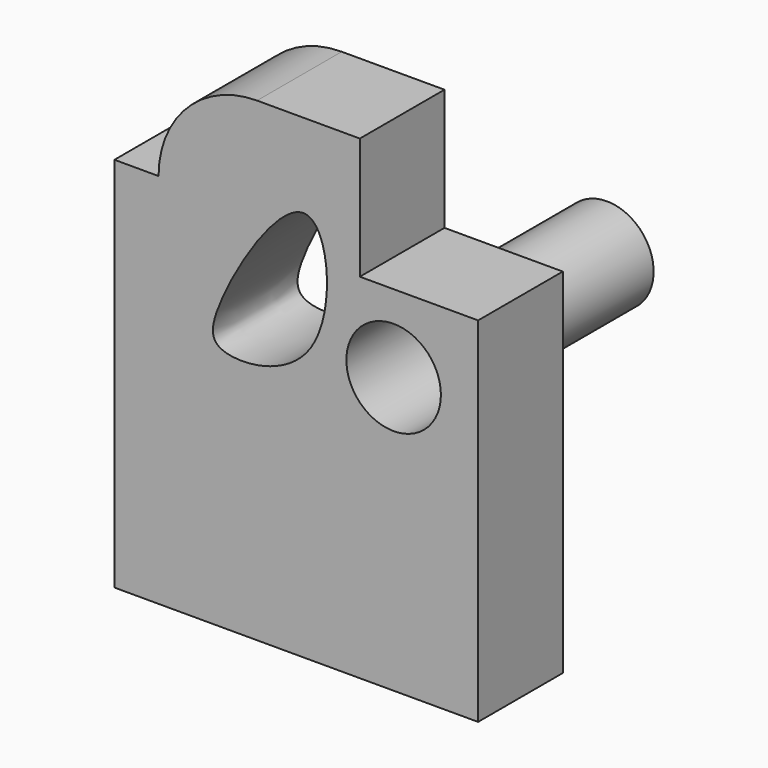
from build123d import *

# Parameters (mm, degrees)
F0_R      = 27.2043930804
F1_DEPTH  = 60.893477872
F2_R      = 56.6833195886
F3_R      = 26.9202980766
F4_DEPTH  = 188.1199926138
F5_DEPTH  = 143.7802445143
F8_DEPTH  = 25.4
F9_DEPTH  = 88.3794147521
F10_DEPTH = 95.6057533622


# Not quite as in the source:
# - a feature of the source that left no trace in its solid (it failed there, or was rolled back) is left out


with BuildPart() as f1:
    # F0 (on Front) → F1 (new body)
    with BuildSketch(Plane.XZ):
        Polygon((-62.7778023481, 114.7176772356), (-62.7778023481, -70.334173739), (121.1167871952, -70.334173739), (121.1167871952, 44.7145961225), (53.0546493828, 44.7145961225), (53.0546493828, 114.7176772356), align=None)
        with Locations((72.5009217858, 0)):
            Circle(F0_R, mode=Mode.SUBTRACT)
        with BuildLine():
            add(Edge.make_bspline(
                [(-29.3809175491, 0), (-21.679578827, 22.4236781976), (31.7086513943, 110.8080219924), (42.4199428526, -16.1208348012), (-30.4596532938, -24.5098615886), (-33.0190651742, -10.5930481079), (-29.3809175491, 0)],
                knots=[0, 0, 0, 0, 0.3160546751, 0.5971945413, 0.8506943264, 1, 1, 1, 1], degree=3))
        make_face(mode=Mode.SUBTRACT)
    extrude(amount=F1_DEPTH)

    # F2
    f2_edges = [f1.edges().sort_by_distance(p)[0] for p in [
        (-62.777802, -30.446739, 114.717677),
    ]]
    fillet(f2_edges, radius=F2_R)

    # F8 (add): a face of the model
    f8_faces = [f1.faces().sort_by_distance(p)[0] for p in [
        (-62.7778023481, -30.446738936, -6.149908046),
    ]]
    extrude(f8_faces, amount=F8_DEPTH)

    # F9 (add): a face of the model
    f9_faces = [f1.faces().sort_by_distance(p)[0] for p in [
        (16.4694924235, -30.446738936, -70.334173739),
    ]]
    extrude(f9_faces, amount=F9_DEPTH)


with BuildPart() as f4:
    # F3 (on face) → F4 (new body)
    with BuildSketch(Plane(origin=(0, 0, 0), x_dir=(-1, 0, 0), z_dir=(0, 1, 0))):
        with Locations((-72.5009217858, 0)):
            Circle(F3_R)
    extrude(amount=F4_DEPTH)

    # F5 (add): a face of the model
    f5_faces = [f4.faces().sort_by_distance(p)[0] for p in [
        (72.5009217858, 188.1199926138, 0),
    ]]
    extrude(f5_faces, amount=-F5_DEPTH)

    # F10 (cut): a face of the model
    f10_faces = [f4.faces().sort_by_distance(p)[0] for p in [
        (72.5009217858, 188.1199926138, 0),
    ]]
    extrude(f10_faces, amount=-F10_DEPTH, mode=Mode.SUBTRACT)


solid = Compound([f1.part, f4.part])
